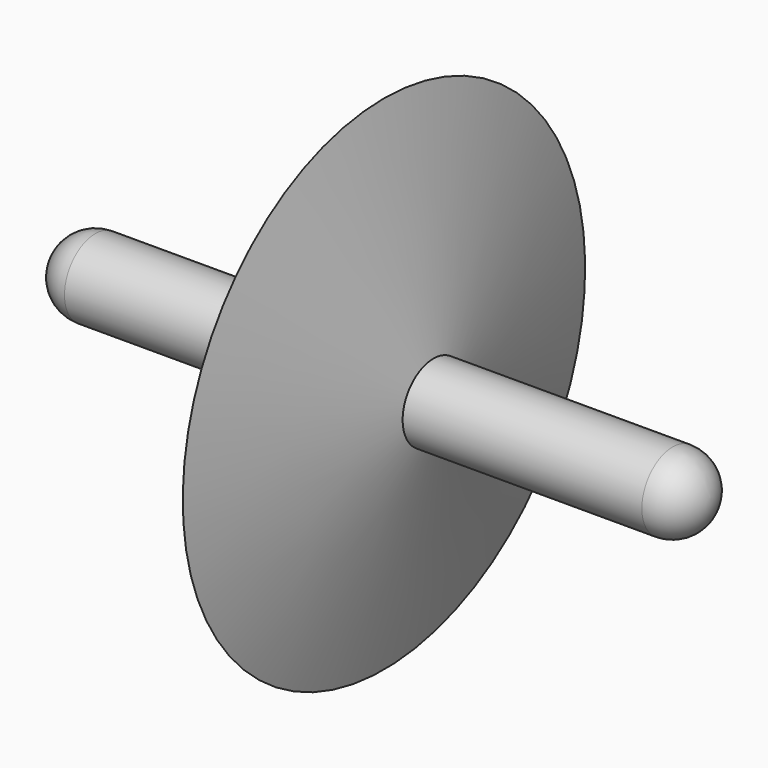
from build123d import *


with BuildPart() as f1:
    # F0 (on Front) → F1 (revolve)
    with BuildSketch(Plane.XZ):
        Polygon((3.2636624089, 2.54), (0, 16.5971969785), (-3.2636624089, 2.54), align=None)
        Polygon((3.2636624089, 2.54), (-3.2636624089, 2.54), (-3.8533747486, 0), (3.8533747486, 0), align=None)
    revolve(axis=Axis((3.749865225, 0, 0), (1, 0, 0)))


with BuildPart() as f3:
    # F0 (on Front) → F3 (revolve)
    with BuildSketch(Plane.XZ):
        with BuildLine():
            ThreePointArc((21.59, 0), (20.8460512242, 1.7960512242), (19.05, 2.54))
            Line((19.05, 2.54), (19.05, 0))
            Line((19.05, 0), (21.59, 0))
        make_face()
        Polygon((19.05, 2.54), (3.2636624089, 2.54), (3.8533747486, 0), (19.05, 0), align=None)
        Polygon((3.2636624089, 2.54), (-3.2636624089, 2.54), (-3.8533747486, 0), (3.8533747486, 0), align=None)
        Polygon((-3.8533747486, 0), (-3.2636624089, 2.54), (-19.05, 2.54), (-19.05, 0), align=None)
        with BuildLine():
            Line((-19.05, 0), (-19.05, 2.54))
            ThreePointArc((-19.05, 2.54), (-20.8460512242, 1.7960512242), (-21.59, 0))
            Line((-21.59, 0), (-19.05, 0))
        make_face()
    revolve(axis=Axis((3.749865225, 0, 0), (1, 0, 0)))

    # F0 (on Front) → F2 (revolve)
    with BuildSketch(Plane.XZ):
        Polygon((3.2636624089, 2.54), (0, 16.5971969785), (-3.2636624089, 2.54), align=None)
    revolve(axis=Axis((3.749865225, 0, 0), (1, 0, 0)))


solid = Compound([f1.part, f3.part])
